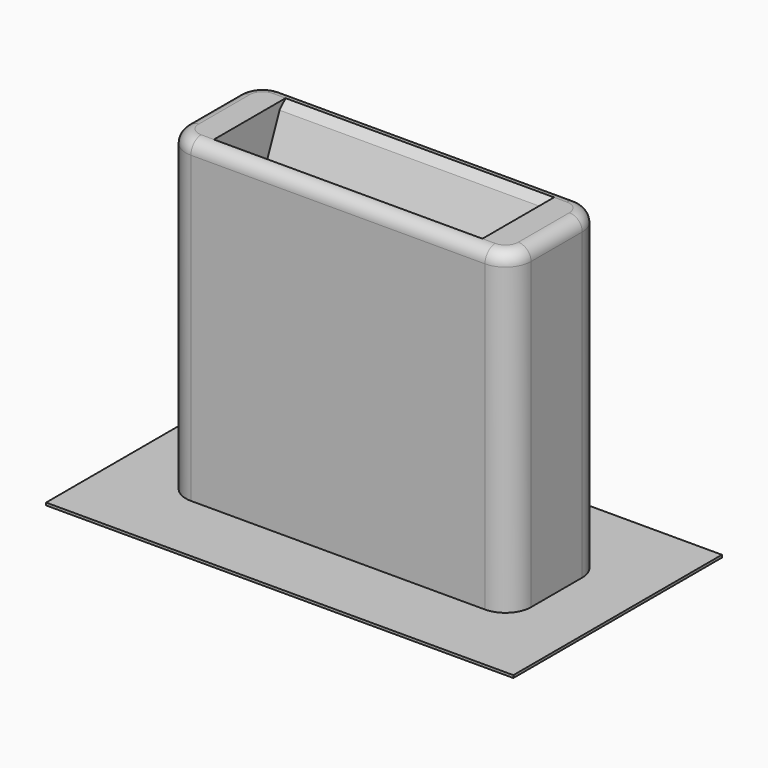
from build123d import *

# Parameters (mm, degrees)
F0_W     = 21
F0_H     = 3
F1_DEPTH = 25
F2_SIZE  = 2
F3_SIZE  = 2
F4_R     = 0.99999
F0_W_2   = 36.543905735
F0_H_2   = 20.3890502453
F5_DEPTH = 0.2


# Not quite as in the source:
# - a fillet or chamfer is up to 0.001 mm smaller than in the source, because OpenCascade refuses the exact size


with BuildPart() as f1:
    # F0 (on Top) → F1 (new body)
    with BuildSketch(Plane.XY):
        with BuildLine():
            Line((-11.5, -4.5), (11.5, -4.5))
            ThreePointArc((11.5, -4.5), (12.9142135624, -3.9142135624), (13.5, -2.5))
            Line((13.5, -2.5), (13.5, 2.5))
            ThreePointArc((13.5, 2.5), (12.9142135624, 3.9142135624), (11.5, 4.5))
            Line((11.5, 4.5), (-11.5, 4.5))
            ThreePointArc((-11.5, 4.5), (-12.9142135624, 3.9142135624), (-13.5, 2.5))
            Line((-13.5, 2.5), (-13.5, -2.5))
            ThreePointArc((-13.5, -2.5), (-12.9142135624, -3.9142135624), (-11.5, -4.5))
        make_face()
        Rectangle(F0_W, F0_H, mode=Mode.SUBTRACT)
    extrude(amount=F1_DEPTH)

    # F2
    f2_edges = [f1.edges().sort_by_distance(p)[0] for p in [
        (0, -1.5, 25),
        (0, 1.5, 25),
        (0, 1.5, 0),
        (0, -1.5, 0),
    ]]
    chamfer(f2_edges, length=F2_SIZE)

    # F3
    f3_edges = [f1.edges().sort_by_distance(p)[0] for p in [
        (0, 1.5, 23),
        (0, -1.5, 23),
        (0, -1.5, 2),
        (0, 1.5, 2),
    ]]
    chamfer(f3_edges, length=F3_SIZE)

    # F4 (radius 1 in the source; OpenCascade refuses exactly that, so slightly less here)
    f4_edges = [f1.edges().sort_by_distance(p)[0] for p in [
        (0, 4.5, 25),
    ]]
    fillet(f4_edges, radius=F4_R)

    # F0 (on Top) → F5 (join)
    with BuildSketch(Plane.XY):
        Rectangle(F0_W_2, F0_H_2)
        with BuildLine():
            ThreePointArc((13.5, -2.5), (12.9142135624, -3.9142135624), (11.5, -4.5))
            Line((11.5, -4.5), (-11.5, -4.5))
            ThreePointArc((-11.5, -4.5), (-12.9142135624, -3.9142135624), (-13.5, -2.5))
            Line((-13.5, -2.5), (-13.5, 2.5))
            ThreePointArc((-13.5, 2.5), (-12.9142135624, 3.9142135624), (-11.5, 4.5))
            Line((-11.5, 4.5), (11.5, 4.5))
            ThreePointArc((11.5, 4.5), (12.9142135624, 3.9142135624), (13.5, 2.5))
            Line((13.5, 2.5), (13.5, -2.5))
        make_face(mode=Mode.SUBTRACT)
    extrude(amount=F5_DEPTH)


solid = f1.part
